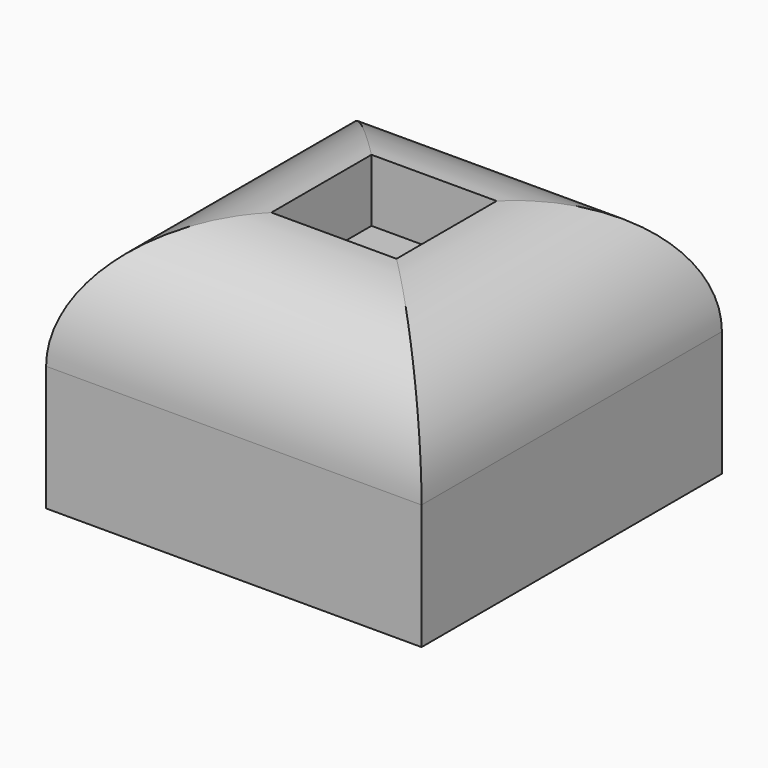
from build123d import *

# Parameters (mm, degrees)
F0_W     = 300
F0_H     = 300
F0_W_2   = 100
F0_H_2   = 100
F1_DEPTH = 200
F2_DEPTH = 150
F3_R     = 99.99999


# Not quite as in the source:
# - a fillet or chamfer is up to 0.001 mm smaller than in the source, because OpenCascade refuses the exact size


with BuildPart() as f1:
    # F0 (on Top) → F1 (new body)
    with BuildSketch(Plane.XY):
        Rectangle(F0_W, F0_H)
        Rectangle(F0_W_2, F0_H_2, mode=Mode.SUBTRACT)
    extrude(amount=F1_DEPTH)

    # F0 (on Top) → F2 (join)
    with BuildSketch(Plane.XY):
        Rectangle(F0_W_2, F0_H_2)
    extrude(amount=F2_DEPTH)

    # F3 (radius 100 in the source; OpenCascade refuses exactly that, so slightly less here)
    f3_edges = [f1.edges().sort_by_distance(p)[0] for p in [
        (-150, 0, 200),
        (0, -150, 200),
        (150, 0, 200),
        (0, 150, 200),
    ]]
    fillet(f3_edges, radius=F3_R)


solid = f1.part
